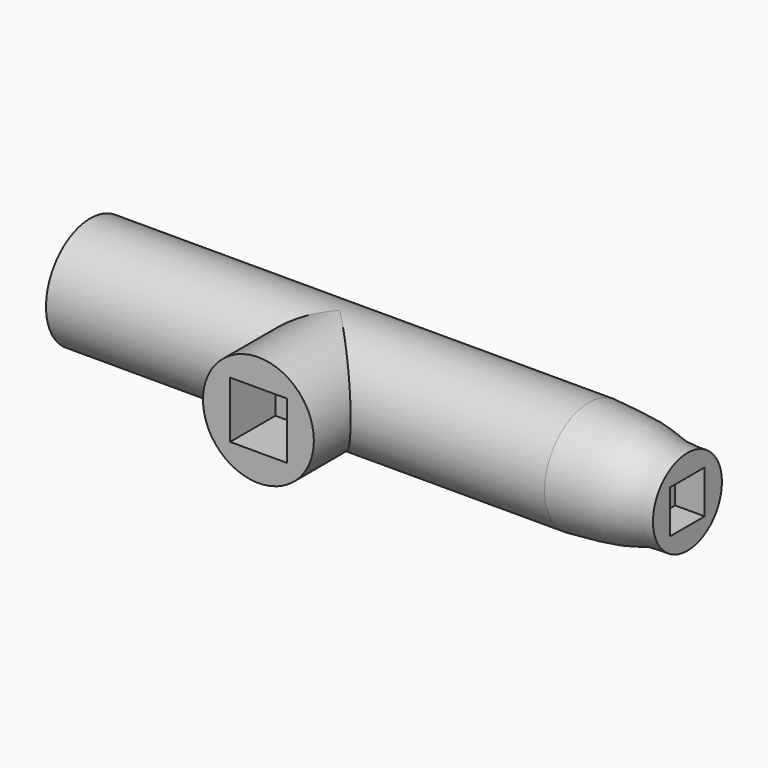
from build123d import *

# Parameters (mm, degrees)
F0_R      = 57.15
F3_DEPTH  = 514.096
F2_R      = 57.15
F5_DEPTH  = 104.648
F6_W      = 58.42
F6_H      = 58.42
F7_DEPTH  = 58.42
F8_W      = 58.42
F8_H      = 58.42
F9_DEPTH  = 58.42
F10_W     = 44.45
F10_H     = 44.45
F11_DEPTH = 30.48


# Not quite as in the source:
# - a feature names something its author has since deleted; it is built from what else it names


with BuildPart() as f3:
    # F0 (on Right) → F3 (new body)
    with BuildSketch(Plane.YZ):
        Circle(F0_R)
    extrude(amount=F3_DEPTH)

    # F1 (on Top) → F4 (revolve)
    with BuildSketch(Plane.XY):
        with BuildLine():
            Line((514.096, 57.15), (514.096, 0))
            Line((514.096, 0), (615.696, 0))
            Line((615.696, 0), (615.696, 44.45))
            add(Edge.make_bspline(
                [(514.096, 57.15), (530.3059150596, 55.8042351211), (558.1923144484, 54.3135523686), (580.3852464856, 48.6501982027), (594.1085406783, 43.9680323111), (608.3163207178, 44.8236773325), (615.696, 44.45)],
                knots=[0, 0, 0, 0, 0.3407026007, 0.5771106283, 0.7657914869, 1, 1, 1, 1], degree=3))
        make_face()
    revolve(axis=Axis((564.896, 0, 0), (-1, 0, 0)))

    # F2 (on Front) → F5 (join)
    with BuildSketch(Plane.XZ):
        with Locations((257.048, 0)):
            Circle(F2_R)
    extrude(amount=F5_DEPTH)

    # F6 (on face) → F7 (cut)
    with BuildSketch(Plane(origin=(0, 0, 0), x_dir=(0, -1, 0), z_dir=(-1, 0, 0))):
        Rectangle(F6_W, F6_H)
    extrude(amount=-F7_DEPTH, mode=Mode.SUBTRACT)

    # F8 (on face) → F9 (cut)
    with BuildSketch(Plane.XZ.offset(104.648)):
        with Locations((257.048, 0)):
            Rectangle(F8_W, F8_H)
    extrude(amount=-F9_DEPTH, mode=Mode.SUBTRACT)

    # F10 (on face) → F11 (cut)
    with BuildSketch(Plane.YZ.offset(615.696)):
        Rectangle(F10_W, F10_H)
    extrude(amount=-F11_DEPTH, mode=Mode.SUBTRACT)


solid = f3.part
